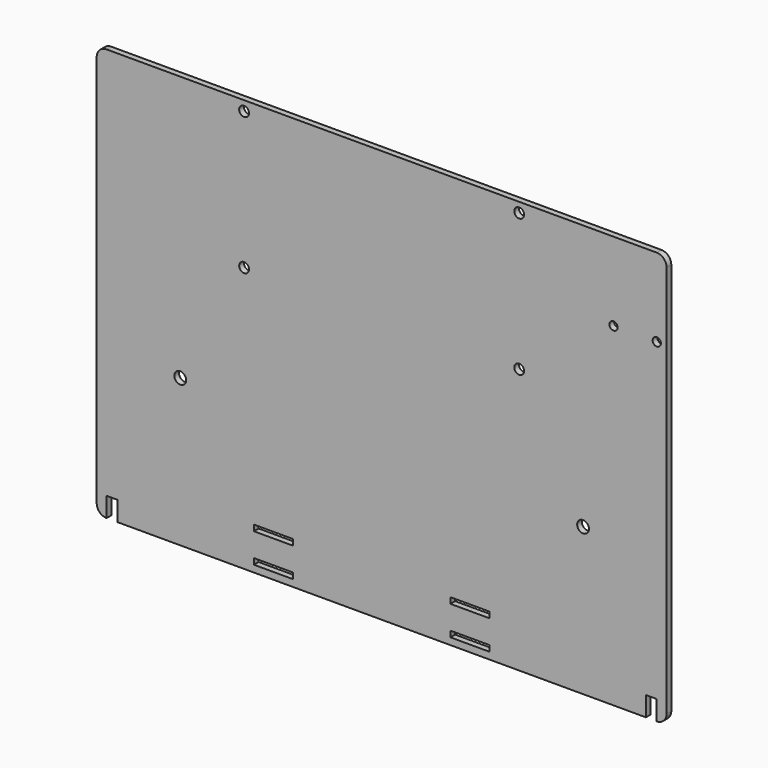
from build123d import *

# Parameters (mm, degrees)
F1_DEPTH = 3
F2_R     = 2.5
F3_DEPTH = 3
F4_R     = 3
F5_DEPTH = 3
F6_R     = 2.1
F7_DEPTH = 3
F8_W     = 20
F8_H     = 3
F9_DEPTH = 3
F10_R    = 4.99999


# Not quite as in the source:
# - a fillet or chamfer is up to 0.001 mm smaller than in the source, because OpenCascade refuses the exact size


with BuildPart() as f1:
    # F0 (on Front) → F1 (new body)
    with BuildSketch(Plane.XZ):
        Polygon((140, -105), (145, -105), (145, 105), (-145, 105), (-145, -105), (-140, -105), (-140, -95), (-134.5, -95), (-134.5, -105), (134.5, -105), (134.5, -95), (140, -95), align=None)
    extrude(amount=F1_DEPTH)

    # F2 (on face) → F3 (cut, through all)
    with BuildSketch(Plane.XZ.offset(3)):
        with Locations((-70, 100)):
            Circle(F2_R)
        with Locations((-70, 30)):
            Circle(F2_R)
        with Locations((70, 100)):
            Circle(F2_R)
        with Locations((70, 30)):
            Circle(F2_R)
    extrude(amount=-F3_DEPTH, mode=Mode.SUBTRACT)

    # F4 (on face) → F5 (cut, through all)
    with BuildSketch(Plane.XZ.offset(3)):
        with Locations((102.5, -30)):
            Circle(F4_R)
        with Locations((-102.5, -30)):
            Circle(F4_R)
    extrude(amount=-F5_DEPTH, mode=Mode.SUBTRACT)

    # F6 (on face) → F7 (cut, through all)
    with BuildSketch(Plane.XZ.offset(3)):
        with Locations((118, 65)):
            Circle(F6_R)
        with Locations((140, 65)):
            Circle(F6_R)
    extrude(amount=-F7_DEPTH, mode=Mode.SUBTRACT)

    # F8 (on face) → F9 (cut, through all)
    with BuildSketch(Plane.XZ.offset(3)):
        with Locations((-55, -85)):
            Rectangle(F8_W, F8_H)
        with Locations((45, -85)):
            Rectangle(F8_W, F8_H)
        with Locations((45, -100)):
            Rectangle(F8_W, F8_H)
        with Locations((-55, -100)):
            Rectangle(F8_W, F8_H)
    extrude(amount=-F9_DEPTH, mode=Mode.SUBTRACT)

    # F10 (radius 5 in the source; OpenCascade refuses exactly that, so slightly less here)
    f10_edges = [f1.edges().sort_by_distance(p)[0] for p in [
        (-145, -1.5, 105),
        (-145, -1.5, -105),
        (145, -1.5, -105),
        (145, -1.5, 105),
    ]]
    fillet(f10_edges, radius=F10_R)


solid = f1.part
